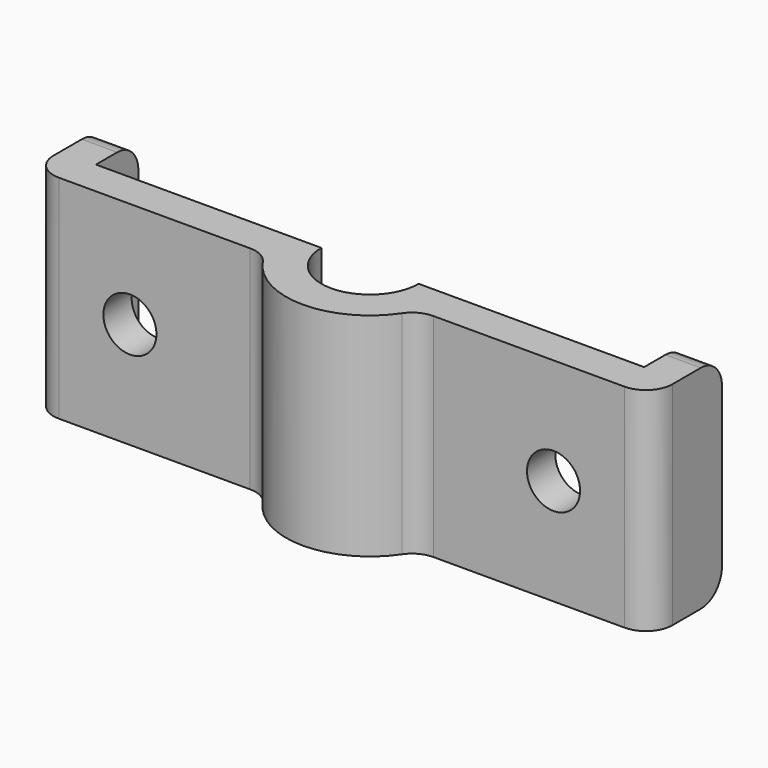
from build123d import *

# Parameters (mm, degrees)
F1_DEPTH = 76.2
F2_R     = 9.525
F4_R     = 9.525
F5_DEPTH = 25.4


with BuildPart() as f1:
    # F0 (on Top) → F1 (new body)
    with BuildSketch(Plane.XY):
        with BuildLine():
            Line((0, 31.75), (0, 0))
            Line((0, 0), (83.7665203959, 0))
            ThreePointArc((83.7665203959, 0), (81.671846117, 6.197067385), (80.9625, 12.7))
            Line((80.9625, 12.7), (12.7, 12.7))
            Line((12.7, 12.7), (12.7, 31.75))
            Line((12.7, 31.75), (0, 31.75))
        make_face()
        with BuildLine():
            ThreePointArc((80.9625, 12.7), (81.671846117, 6.197067385), (83.7665203959, 0))
            Line((83.7665203959, 0), (99.139637834, 0))
            ThreePointArc((99.139637834, 0), (95.0901427653, 5.7846359667), (93.6625, 12.7))
            Line((93.6625, 12.7), (80.9625, 12.7))
        make_face()
        with BuildLine():
            Line((99.139637834, 0), (83.7665203959, 0))
            ThreePointArc((83.7665203959, 0), (111.125, -17.4625), (138.4834796041, 0))
            Line((138.4834796041, 0), (123.110362166, 0))
            ThreePointArc((123.110362166, 0), (111.125, -4.7625), (99.139637834, 0))
        make_face()
        with BuildLine():
            ThreePointArc((141.2875, 12.7), (140.578153883, 6.197067385), (138.4834796041, 0))
            Line((138.4834796041, 0), (222.25, 0))
            Line((222.25, 0), (222.25, 31.75))
            Line((222.25, 31.75), (209.55, 31.75))
            Line((209.55, 31.75), (209.55, 12.7))
            Line((209.55, 12.7), (141.2875, 12.7))
        make_face()
        with BuildLine():
            Line((123.110362166, 0), (138.4834796041, 0))
            ThreePointArc((138.4834796041, 0), (140.578153883, 6.197067385), (141.2875, 12.7))
            Line((141.2875, 12.7), (128.5875, 12.7))
            ThreePointArc((128.5875, 12.7), (127.1598572347, 5.7846359667), (123.110362166, 0))
        make_face()
    extrude(amount=F1_DEPTH)

    # F2
    f2_edges = [f1.edges().sort_by_distance(p)[0] for p in [
        (0, 0, 38.1),
        (6.35, 31.75, 76.2),
        (215.9, 31.75, 76.2),
        (215.9, 31.75, 0),
        (6.35, 31.75, 0),
        (138.48348, 0, 38.1),
        (83.76652, 0, 38.1),
        (222.25, 0, 38.1),
    ]]
    fillet(f2_edges, radius=F2_R)

    # F4 (on face) + F3 (on face) → F5 (cut)
    with BuildSketch(Plane.XZ):
        with Locations((35.0641996562, 38.1)):
            Circle(F4_R)
    with BuildSketch(Plane.XZ):
        with BuildLine():
            ThreePointArc((196.7108003438, 38.1), (187.1858003438, 47.625), (177.6608003438, 38.1))
            ThreePointArc((177.6608003438, 38.1), (187.1858003438, 28.575), (196.7108003438, 38.1))
        make_face()
    extrude(amount=-F5_DEPTH, mode=Mode.SUBTRACT)


solid = f1.part
